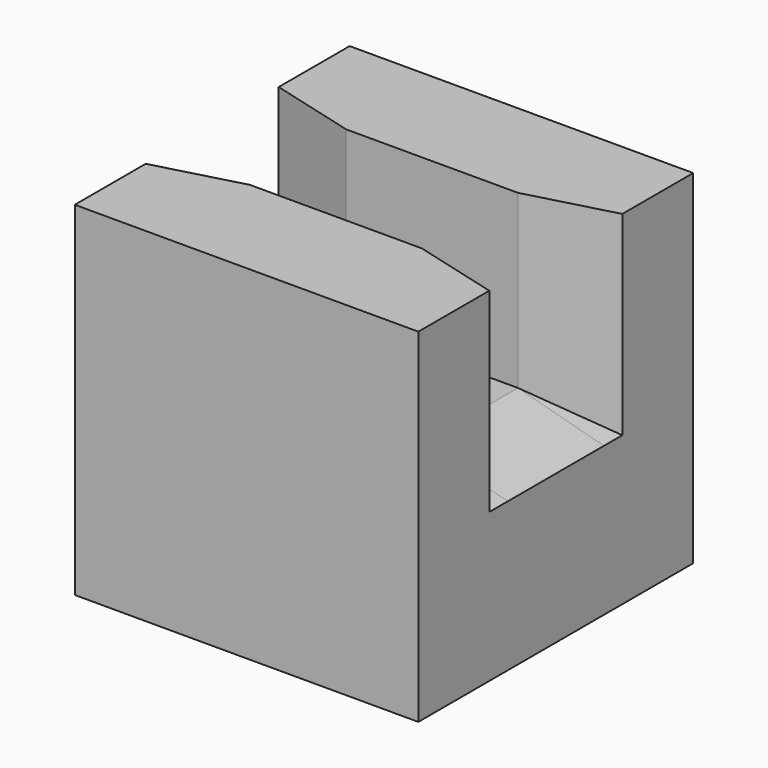
from build123d import *

# Parameters (mm, degrees)
F0_W     = 40
F0_H     = 40
F1_DEPTH = 40
F4_DEPTH = 7
F6_REACH = 50.3537618041
F8_REACH = 50.3537618041


with BuildPart() as f1:
    # F0 (on Front) → F1 (new body)
    with BuildSketch(Plane.XZ):
        with Locations((20, 20)):
            Rectangle(F0_W, F0_H)
    extrude(amount=F1_DEPTH)

    # F3 (on offset) → F4 (cut, symmetric)
    with BuildSketch(Plane.XZ.offset(20)):
        Polygon((0, 40), (0, 17.3205080757), (10, 20), (30, 20), (40, 17.3205080757), (40, 40), align=None)
    extrude(amount=F4_DEPTH, both=True, mode=Mode.SUBTRACT)

    f6_end = Plane(origin=(5, -20, 18.6602540378), x_dir=(0.9659258263, 0, 0.2588190451), z_dir=(-0.2588190451, 0, 0.9659258263))
    # F5 (on face) → F6 (cut, up to a plane its end follows)
    with BuildSketch(Plane.XY.offset(40)):
        Polygon((10, -13), (0, -10.3205080757), (0, -13), align=None)
        Polygon((0, -27), (0, -29.6794919243), (10, -27), align=None)
    f6_long = extrude(amount=-F6_REACH, mode=Mode.PRIVATE)
    add(split(f6_long, bisect_by=f6_end, keep=Keep.TOP, mode=Mode.PRIVATE), mode=Mode.SUBTRACT)

    f8_end = Plane(origin=(35, -20, 18.6602540378), x_dir=(0.9659258263, 0, -0.2588190451), z_dir=(0.2588190451, 0, 0.9659258263))
    # F7 (on face) → F8 (cut, up to a plane its end follows)
    with BuildSketch(Plane.XY.offset(40)):
        Polygon((40, -10.3205080757), (30, -13), (40, -13), align=None)
        Polygon((40, -27), (30, -27), (40, -29.6794919243), align=None)
    f8_long = extrude(amount=-F8_REACH, mode=Mode.PRIVATE)
    add(split(f8_long, bisect_by=f8_end, keep=Keep.TOP, mode=Mode.PRIVATE), mode=Mode.SUBTRACT)


solid = f1.part
